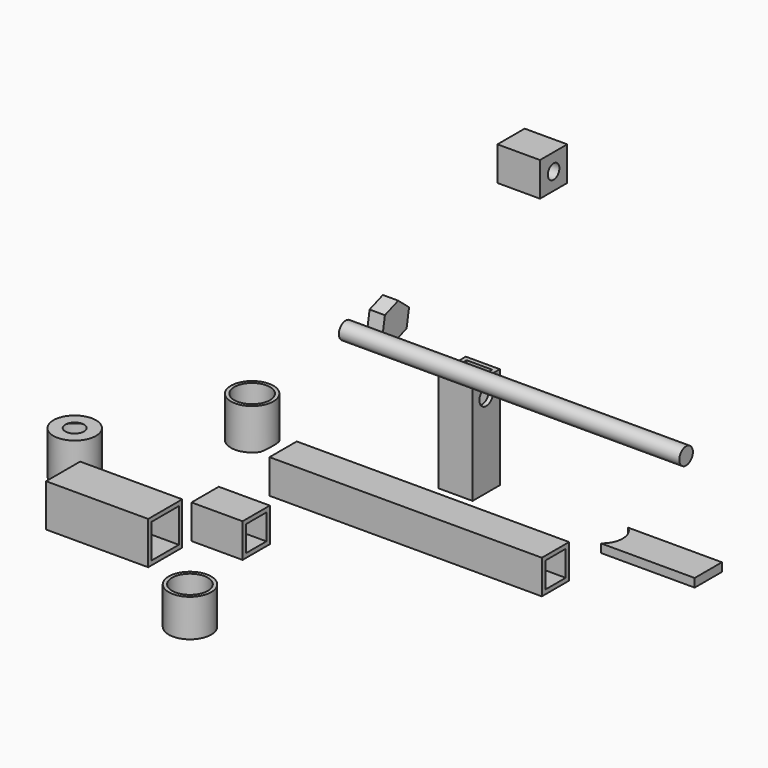
from build123d import *

# Parameters (mm, degrees)
F0_W      = 160
F0_H      = 20
F1_DEPTH  = 10
F2_W      = 25
F2_H      = 25
F2_W_2    = 20
F2_H_2    = 20
F3_DEPTH  = 60
F4_W      = 15
F4_H      = 15
F5_DEPTH  = 160
F6_W      = 20
F6_H      = 20
F6_W_2    = 15
F6_H_2    = 15
F7_DEPTH  = 30
F8_R      = 12.5
F8_R_2    = 10.5
F9_DEPTH  = 22
F10_R     = 12.5
F10_R_2   = 10.5
F11_DEPTH = 24
F12_R     = 12.5
F13_DEPTH = 25
F14_D     = 21
F14_DEPTH = 22
F14_TIP   = 6.3090364998
F15_W     = 55
F15_H     = 20
F16_DEPTH = 5
F17_W     = 20
F17_H     = 60
F17_R     = 5
F18_DEPTH = 20
F19_W     = 20
F19_H     = 20
F20_DEPTH = 25
F21_D     = 8.5
F22_R     = 5
F23_DEPTH = 200
F25_DEPTH = 9
F27_DEPTH = 25
F29_DEPTH = 25
F30_R     = 10.5
F31_DEPTH = 2
F32_W     = 15
F32_H     = 15
F33_DEPTH = 60
F34_R     = 12.75
F35_DEPTH = 5


# Not quite as in the source:
# - a feature names something its author has since deleted; it is built from what else it names


with BuildPart() as f1:
    # F0 (on Front) → F1 (new body, symmetric)
    with BuildSketch(Plane.XZ):
        with Locations((80, 0)):
            Rectangle(F0_W, F0_H)
    extrude(amount=F1_DEPTH, both=True)

    # F4 (on Right) → F5 (cut)
    with BuildSketch(Plane.YZ):
        Rectangle(F4_W, F4_H)
    extrude(amount=F5_DEPTH, mode=Mode.SUBTRACT)


with BuildPart() as f3:
    # F2 (on Right) → F3 (new body)
    with BuildSketch(Plane.YZ):
        with Locations((-161.6110950708, 51.756149815)):
            Rectangle(F2_W, F2_H)
        with Locations((-161.6110950708, 51.756149815)):
            Rectangle(F2_W_2, F2_H_2, mode=Mode.SUBTRACT)
    extrude(amount=F3_DEPTH)


with BuildPart() as f7:
    # F6 (on Right) → F7 (new body)
    with BuildSketch(Plane.YZ):
        with Locations((-57.3030114174, -0.1235169003)):
            Rectangle(F6_W, F6_H)
        with Locations((-57.3030114174, -0.1235169003)):
            Rectangle(F6_W_2, F6_H_2, mode=Mode.SUBTRACT)
    extrude(amount=F7_DEPTH)


with BuildPart() as f9:
    # F8 (on Top) → F9 (new body)
    with BuildSketch(Plane.XY):
        with Locations((38.4034886956, -116.4533868432)):
            Circle(F8_R)
        with Locations((38.4034886956, -116.4533868432)):
            Circle(F8_R_2, mode=Mode.SUBTRACT)
    extrude(amount=-F9_DEPTH)


with BuildPart() as f11:
    # F10 (on Top) → F11 (new body)
    with BuildSketch(Plane.XY):
        with Locations((-28.8939643651, 13.3474841714)):
            Circle(F10_R)
        with Locations((-28.8939643651, 13.3474841714)):
            Circle(F10_R_2, mode=Mode.SUBTRACT)
    extrude(amount=F11_DEPTH)

    # F26 (on Front) → F27 (cut)
    with BuildSketch(Plane.XZ):
        Polygon((-18.3939643651, 0), (-16.3939643651, 0), (-16.3939643651, 1.1547005384), align=None)
    extrude(amount=-F27_DEPTH, mode=Mode.SUBTRACT)

    # F28 (on Front) → F29 (cut)
    with BuildSketch(Plane.XZ):
        Polygon((-41.3939643651, 1.1547005384), (-41.3939643651, 0), (-39.3939643651, 0), align=None)
    extrude(amount=-F29_DEPTH, mode=Mode.SUBTRACT)


with BuildPart() as f13:
    # F12 (on Top) → F13 (new body)
    with BuildSketch(Plane.XY):
        with Locations((-69.8703065715, -65.7545542214)):
            Circle(F12_R)
    extrude(amount=F13_DEPTH)

    # F14
    with Locations(Plane(origin=(0, 0, 0), x_dir=(1, 0, 0), z_dir=(0, 0, -1))):
        with Locations((-69.8703065715, 65.7545542214)):
            Hole(F14_D / 2, depth=F14_DEPTH)
            with Locations((0, 0, -(F14_DEPTH + F14_TIP / 2))):  # 118° drill point
                Cone(0, F14_D / 2, F14_TIP, mode=Mode.SUBTRACT)


with BuildPart() as f16:
    # F15 (on face) → F16 (new body)
    with BuildSketch(Plane(origin=(0, 0, -10), x_dir=(1, 0, 0), z_dir=(0, 0, -1))):
        with Locations((175.8168041706, -58.102128388)):
            Rectangle(F15_W, F15_H)
    extrude(amount=F16_DEPTH)

    # F34 (on face) → F35 (cut)
    with BuildSketch(Plane(origin=(0, 0, -10), x_dir=(1, 0, 0), z_dir=(0, 0, -1))):
        with Locations((140.3318259962, -58.0808729371)):
            Circle(F34_R)
    extrude(amount=F35_DEPTH, mode=Mode.SUBTRACT)


with BuildPart() as f18:
    # F17 (on Right) → F18 (new body)
    with BuildSketch(Plane.YZ):
        with Locations((124.1480589582, -26.6051380336)):
            Rectangle(F17_W, F17_H)
        with Locations((124.1480589582, -6.6051380336)):
            Circle(F17_R, mode=Mode.SUBTRACT)
    extrude(amount=F18_DEPTH)

    # F32 (on face) → F33 (cut)
    with BuildSketch(Plane.XY.offset(3.3948619664)):
        with Locations((10.0230817938, 124.0749582648)):
            Rectangle(F32_W, F32_H)
    extrude(amount=-F33_DEPTH, mode=Mode.SUBTRACT)


with BuildPart() as f20:
    # F19 (on Right) → F20 (new body)
    with BuildSketch(Plane.YZ):
        with Locations((167.3894077539, 93.7553744961)):
            Rectangle(F19_W, F19_H)
    extrude(amount=F20_DEPTH)

    # F21 (through all)
    with Locations(Plane(origin=(0, 0, 0), x_dir=(0, 1, 0), z_dir=(-1, 0, 0))):
        with Locations((167.3894077539, -93.7553744961)):
            Hole(F21_D / 2)


with BuildPart() as f23:
    # F22 (on Right) → F23 (new body)
    with BuildSketch(Plane.YZ):
        with Locations((45.9281019866, 52.9470965266)):
            Circle(F22_R)
    extrude(amount=F23_DEPTH)


with BuildPart() as f25:
    # F24 (on Right) → F25 (new body)
    with BuildSketch(Plane.YZ):
        Polygon((79.4154354066, 43.138094305), (81.2119157193, 53.3739459299), (73.2456483392, 60.0476693305), (63.4829006463, 56.4855411063), (61.6864203336, 46.2496894814), (69.6526877137, 39.5759660808), align=None)
    extrude(amount=F25_DEPTH)


with BuildPart() as f31:
    # F30 (on Top) → F31 (new body)
    with BuildSketch(Plane.XY):
        with Locations((-28.7946469224, 13.378466991)):
            Circle(F30_R)
    extrude(amount=F31_DEPTH)


solid = Compound([f1.part, f3.part, f7.part, f9.part, f11.part, f13.part, f16.part, f18.part, f20.part, f23.part, f25.part, f31.part])
